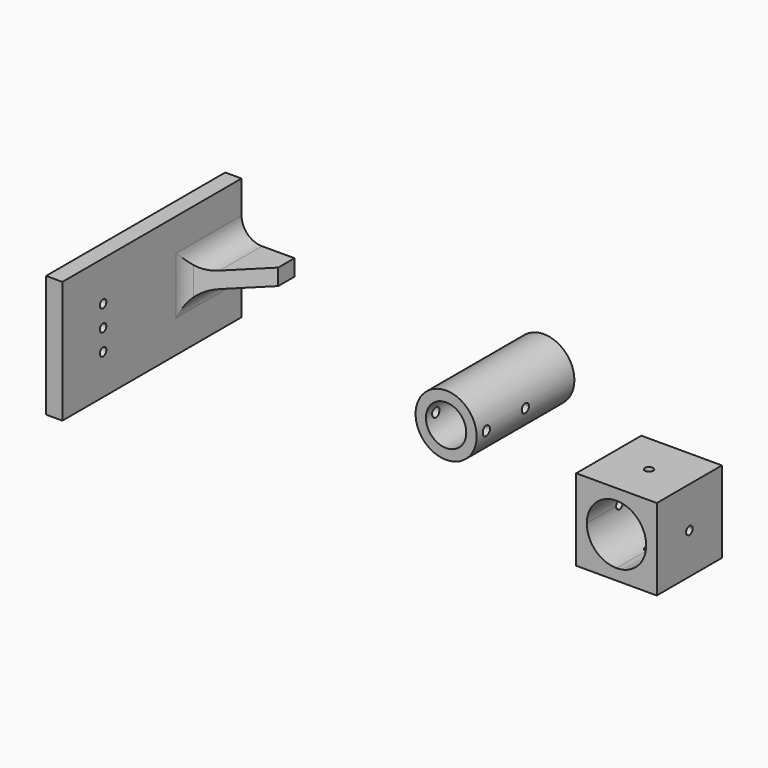
from build123d import *

# Parameters (mm, degrees)
F0_R         = 7.5
F0_R_2       = 4.95
F1_DEPTH     = 30
F4_DEPTH     = 25
F6_DEPTH     = 20
F8_DEPTH     = 21
F10_DEPTH    = 21
F11_W        = 30
F11_H        = 30
F12_DEPTH    = 4
F13_W        = 4
F13_H        = 13
F14_DEPTH    = 25
F15_DEPTH    = 30
F16_DEPTH    = 30
F18_DEPTH    = 5
F19_T4_DEPTH = 132.5841493983
F20_R        = 5
F22_DEPTH    = 5


# Not quite as in the source:
# - a fillet or chamfer that OpenCascade refuses, or shapes differently, is made with other operations: its cross-section is extruded or revolved along the edge and cut away or added


with BuildPart() as f1:
    # F0 (on Front) → F1 (new body)
    with BuildSketch(Plane.XZ):
        Circle(F0_R)
        Circle(F0_R_2, mode=Mode.SUBTRACT)
    extrude(amount=-F1_DEPTH)

    # F3 (on offset) → F4 (cut)
    with BuildSketch(Plane.YZ.offset(7.5)):
        with BuildLine():
            Line((1.8706106639, 0), (2.9919834342, 0))
            Line((2.9919834342, 0), (4.1133562045, 0))
            ThreePointArc((4.1133562045, 0), (2.9919834342, 1.1213727703), (1.8706106639, 0))
        make_face()
        with BuildLine():
            Line((4.1133562045, 0), (2.9919834342, 0))
            Line((2.9919834342, 0), (1.8706106639, 0))
            ThreePointArc((1.8706106639, 0), (2.9919834342, -1.1213727703), (4.1133562045, 0))
        make_face()
        with BuildLine():
            ThreePointArc((14.9805936962, 1.0938833623), (14.2071013529, 0.7734923433), (13.8867103339, 0))
            Line((13.8867103339, 0), (14.9805936962, 0))
            Line((14.9805936962, 0), (14.9805936962, 1.0938833623))
        make_face()
        with BuildLine():
            Line((14.9805936962, 0), (13.8867103339, 0))
            ThreePointArc((13.8867103339, 0), (14.9805936962, -1.0938833623), (16.0744770585, 0))
            Line((16.0744770585, 0), (14.9805936962, 0))
        make_face()
        with BuildLine():
            Line((14.9805936962, 1.0938833623), (14.9805936962, 0))
            Line((14.9805936962, 0), (16.0744770585, 0))
            ThreePointArc((16.0744770585, 0), (15.7540860395, 0.7734923433), (14.9805936962, 1.0938833623))
        make_face()
    extrude(amount=-F4_DEPTH, mode=Mode.SUBTRACT)


with BuildPart() as f6:
    # F5 (on Front) → F6 (new body)
    with BuildSketch(Plane.XZ):
        with BuildLine():
            Line((41.8351665139, 0), (31.9413468242, 0))
            Line((31.9413468242, 0), (31.9413468242, -10))
            Line((31.9413468242, -10), (34.5435520147, -10))
            ThreePointArc((34.5435520147, -10), (36.6792164557, -4.8440499418), (41.8351665139, -2.7083855008))
            Line((41.8351665139, -2.7083855008), (41.8351665139, 0))
        make_face()
        with BuildLine():
            Line((51.7289862037, 0), (41.8351665139, 0))
            Line((41.8351665139, 0), (41.8351665139, -2.7083855008))
            ThreePointArc((41.8351665139, -2.7083855008), (46.9911165721, -4.8440499418), (49.1267810131, -10))
            Line((49.1267810131, -10), (51.7289862037, -10))
            Line((51.7289862037, -10), (51.7289862037, 0))
        make_face()
        with BuildLine():
            Line((51.7289862037, -20), (51.7289862037, -10))
            Line((51.7289862037, -10), (49.1267810131, -10))
            ThreePointArc((49.1267810131, -10), (46.9911165721, -15.1559500582), (41.8351665139, -17.2916144992))
            Line((41.8351665139, -17.2916144992), (41.8351665139, -20))
            Line((41.8351665139, -20), (51.7289862037, -20))
        make_face()
        with BuildLine():
            Line((34.5435520147, -10), (31.9413468242, -10))
            Line((31.9413468242, -10), (31.9413468242, -20))
            Line((31.9413468242, -20), (41.8351665139, -20))
            Line((41.8351665139, -20), (41.8351665139, -17.2916144992))
            ThreePointArc((41.8351665139, -17.2916144992), (36.6792164557, -15.1559500582), (34.5435520147, -10))
        make_face()
    extrude(amount=-F6_DEPTH)

    # F7 (on face) → F8 (cut)
    with BuildSketch(Plane.YZ.offset(51.7289862037)):
        with BuildLine():
            ThreePointArc((11, -10), (10.7071067812, -9.2928932188), (10, -9))
            Line((10, -9), (10, -11))
            ThreePointArc((10, -11), (10.7071067812, -10.7071067812), (11, -10))
        make_face()
        with BuildLine():
            Line((10, -11), (10, -9))
            ThreePointArc((10, -9), (9, -10), (10, -11))
        make_face()
    extrude(amount=-F8_DEPTH, mode=Mode.SUBTRACT)

    # F9 (on face) → F10 (cut)
    with BuildSketch(Plane.XY):
        with BuildLine():
            ThreePointArc((42.8351665139, 10), (42.5422732951, 10.7071067812), (41.8351665139, 11))
            Line((41.8351665139, 11), (41.8351665139, 9))
            ThreePointArc((41.8351665139, 9), (42.5422732951, 9.2928932188), (42.8351665139, 10))
        make_face()
        with BuildLine():
            Line((41.8351665139, 9), (41.8351665139, 11))
            ThreePointArc((41.8351665139, 11), (40.8351665139, 10), (41.8351665139, 9))
        make_face()
    extrude(amount=-F10_DEPTH, mode=Mode.SUBTRACT)


with BuildPart() as f12:
    # F11 (on Top) → F12 (new body)
    with BuildSketch(Plane.XY):
        with Locations((-76.2343985998, 15)):
            Rectangle(F11_W, F11_H)
    extrude(amount=F12_DEPTH)

    # F13 (on face) → F14 (join)
    with BuildSketch(Plane.XZ):
        with Locations((-76.2343985998, -6.5)):
            Rectangle(F13_W, F13_H)
        Polygon((-74.4660645723, 4), (-78.2343985998, 4), (-78.2343985998, 0), (-74.2343985998, 0), (-74.2343985998, 4), align=None)
        Polygon((-78.2343985998, 17), (-78.2343985998, 4), (-74.4660645723, 4), (-74.2343985998, 4), (-74.2343985998, 17), align=None)
    extrude(amount=F14_DEPTH)

    # F15 (add): a face of the model
    f15_faces = [f12.faces().sort_by_distance(p)[0] for p in [
        (-76.2343985998, 0, -6.5),
    ]]
    extrude(f15_faces, amount=F15_DEPTH)

    # F16 (add): a face of the model
    f16_faces = [f12.faces().sort_by_distance(p)[0] for p in [
        (-76.2343985998, 0, 10.5),
    ]]
    extrude(f16_faces, amount=F16_DEPTH)

    # F17 (on face) → F18 (cut)
    with BuildSketch(Plane(origin=(-78.2343985998, 0, 0), x_dir=(0, -1, 0), z_dir=(-1, 0, 0))):
        with BuildLine():
            ThreePointArc((12.5, 1), (13.2071067812, 1.2928932188), (13.5, 2))
            Line((13.5, 2), (12.5, 2))
            Line((12.5, 2), (12.5, 1))
        make_face()
        with BuildLine():
            Line((12.5, 2), (13.5, 2))
            ThreePointArc((13.5, 2), (13.2071067812, 2.7071067812), (12.5, 3))
            Line((12.5, 3), (12.5, 2))
        make_face()
        with BuildLine():
            ThreePointArc((13.5, -3.2), (13.2071067812, -2.4928932188), (12.5, -2.2))
            ThreePointArc((12.5, -2.2), (11.7928932188, -3.9071067812), (13.5, -3.2))
        make_face()
        with BuildLine():
            ThreePointArc((13.5, 7.2002243251), (11.7928932188, 7.9073311062), (12.5, 6.2002243251))
            ThreePointArc((12.5, 6.2002243251), (13.2071067812, 6.4931175439), (13.5, 7.2002243251))
        make_face()
        with BuildLine():
            Line((12.5, 1), (12.5, 2))
            Line((12.5, 2), (11.5, 2))
            ThreePointArc((11.5, 2), (11.7928932188, 1.2928932188), (12.5, 1))
        make_face()
        with BuildLine():
            Line((11.5, 2), (12.5, 2))
            Line((12.5, 2), (12.5, 3))
            ThreePointArc((12.5, 3), (11.7928932188, 2.7071067812), (11.5, 2))
        make_face()
    extrude(amount=-F18_DEPTH, mode=Mode.SUBTRACT)

    # F19: chamfer of 25 on 1 edges, made by hand


with BuildPart() as f19_tool2:
    # F19_s3 → F19_t4 (new body)
    with BuildSketch(Plane.XY.offset(-64.2920746991)):
        Polygon((-61.2343985998, 25), (-86.2343985998, 0), (-61.2343985998, 0), align=None)
    extrude(amount=F19_T4_DEPTH)

    split(bisect_by=Plane.YZ.offset(-74.2343985998), keep=Keep.TOP)


with BuildPart() as f12_1:
    add(f12.part)

    # F19_t1: cut F19_tool2
    add(f19_tool2.part, mode=Mode.SUBTRACT)

    # F20
    f20_edges = [f12_1.edges().sort_by_distance(p)[0] for p in [
        (-74.234399, 12, 2),
        (-74.234399, 21, 0),
        (-74.234399, 21, 4),
    ]]
    fillet(f20_edges, radius=F20_R)

    # F21 (on face) → F22 (cut)
    with BuildSketch(Plane(origin=(0, 0, 0), x_dir=(1, 0, 0), z_dir=(0, 0, -1))):
        with BuildLine():
            ThreePointArc((-84.7343985998, -24), (-85.7343985998, -25), (-84.7343985998, -26))
            Line((-84.7343985998, -26), (-84.7343985998, -24))
        make_face()
        with BuildLine():
            Line((-84.7343985998, -24), (-84.7343985998, -26))
            ThreePointArc((-84.7343985998, -26), (-84.0272918186, -25.7071067812), (-83.7343985998, -25))
            ThreePointArc((-83.7343985998, -25), (-84.0272918186, -24.2928932188), (-84.7343985998, -24))
        make_face()
        with BuildLine():
            ThreePointArc((-84.7343985998, -18.8739860207), (-85.7343985998, -19.8739860207), (-84.7343985998, -20.8739860207))
            Line((-84.7343985998, -20.8739860207), (-84.7343985998, -18.8739860207))
        make_face()
        with BuildLine():
            Line((-84.7343985998, -18.8739860207), (-84.7343985998, -20.8739860207))
            ThreePointArc((-84.7343985998, -20.8739860207), (-84.0272918186, -20.5810928019), (-83.7343985998, -19.8739860207))
            ThreePointArc((-83.7343985998, -19.8739860207), (-84.0272918186, -19.1668792395), (-84.7343985998, -18.8739860207))
        make_face()
        with BuildLine():
            ThreePointArc((-84.7343985998, -13.8739860207), (-85.7343985998, -14.8739860207), (-84.7343985998, -15.8739860207))
            Line((-84.7343985998, -15.8739860207), (-84.7343985998, -13.8739860207))
        make_face()
        with BuildLine():
            Line((-84.7343985998, -13.8739860207), (-84.7343985998, -15.8739860207))
            ThreePointArc((-84.7343985998, -15.8739860207), (-84.0272918186, -15.5810928019), (-83.7343985998, -14.8739860207))
            ThreePointArc((-83.7343985998, -14.8739860207), (-84.0272918186, -14.1668792395), (-84.7343985998, -13.8739860207))
        make_face()
        with BuildLine():
            Line((-84.7343985998, -11.3524029255), (-84.7343985998, -9.3524029255))
            ThreePointArc((-84.7343985998, -9.3524029255), (-85.7343985998, -10.3524029255), (-84.7343985998, -11.3524029255))
        make_face()
        with BuildLine():
            ThreePointArc((-83.7343985998, -10.3524029255), (-84.0272918186, -9.6452961443), (-84.7343985998, -9.3524029255))
            Line((-84.7343985998, -9.3524029255), (-84.7343985998, -11.3524029255))
            ThreePointArc((-84.7343985998, -11.3524029255), (-84.0272918186, -11.0595097067), (-83.7343985998, -10.3524029255))
        make_face()
    extrude(amount=-F22_DEPTH, mode=Mode.SUBTRACT)


solid = Compound([f1.part, f6.part, f12_1.part])
